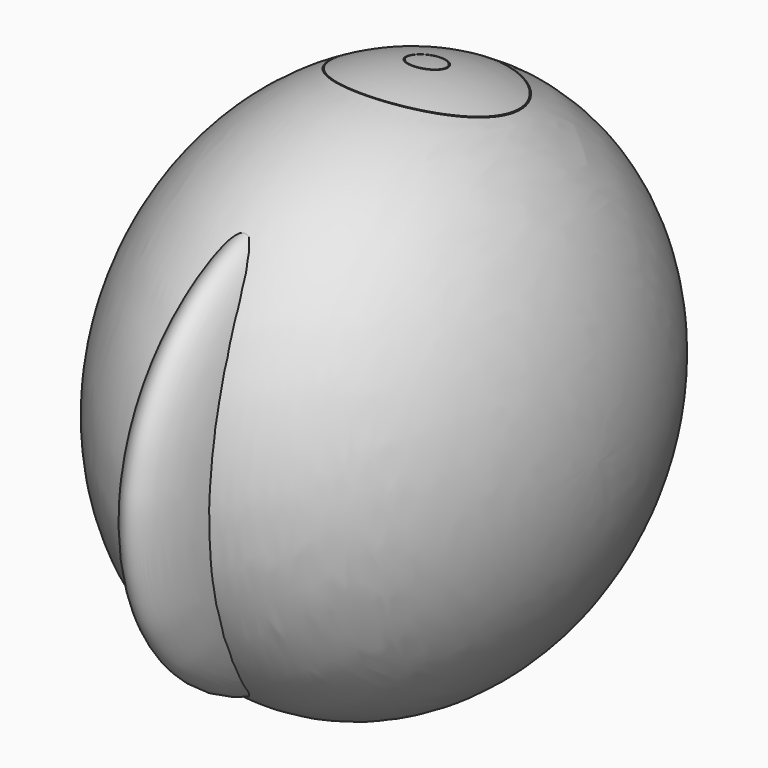
from build123d import *

# Parameters (mm, degrees)
F6_DEPTH = 250.0010001


with BuildPart() as f1:
    # F0 (on Top) → F1 (revolve)
    with BuildSketch(Plane.XY):
        with BuildLine():
            Line((0, 0), (50, 0))
            add(Edge.make_bspline(
                [(50, 0), (50, 200), (0, 200)],
                knots=[1.5707963268, 1.5707963268, 1.5707963268, 3.1415926536, 3.1415926536, 3.1415926536], degree=2, weights=[1, 0.7071067812, 1]))
            Line((0, 200), (0, 0))
        make_face()
        with BuildLine():
            Line((0, 0), (0, 200))
            add(Edge.make_bspline(
                [(0, 200), (-50, 200), (-50, 0)],
                knots=[3.1415926536, 3.1415926536, 3.1415926536, 4.7123889804, 4.7123889804, 4.7123889804], degree=2, weights=[1, 0.7071067812, 1]))
            Line((-50, 0), (0, 0))
        make_face()
    revolve(axis=Axis((53.4832403064, 0, 0), (1, 0, 0)))


with BuildPart() as f3:
    # F2 (on Top) → F3 (revolve)
    with BuildSketch(Plane.XY):
        with BuildLine():
            Line((0, 100), (200, 100))
            add(Edge.make_bspline(
                [(200, 100), (200, 350), (0, 350), (-200, 350), (-200, 100)],
                knots=[4.7123889804, 4.7123889804, 4.7123889804, 6.2831853072, 6.2831853072, 7.853981634, 7.853981634, 7.853981634], degree=2, weights=[1, 0.7071067812, 1, 0.7071067812, 1]))
            Line((-200, 100), (-175.48173666, 100))
            Line((-175.48173666, 100), (0, 100))
        make_face()
    revolve(axis=Axis((253.5901129246, 100, 0), (1, 0, 0)))


with BuildPart() as f6_tool:
    # F5 (on Top) → F6 (new body, through all)
    with BuildSketch(Plane.XY):
        with BuildLine():
            ThreePointArc((0, 226), (-76, 150), (0, 74))
            Line((0, 74), (0, 75))
            ThreePointArc((0, 75), (-75, 150), (0, 225))
            Line((0, 225), (0, 226))
        make_face()
        with BuildLine():
            Line((0, 75), (0, 74))
            ThreePointArc((0, 74), (53.7401153702, 96.2598846298), (76, 150))
            ThreePointArc((76, 150), (53.7401153702, 203.7401153702), (0, 226))
            Line((0, 226), (0, 225))
            ThreePointArc((0, 225), (53.033008589, 203.033008589), (75, 150))
            ThreePointArc((75, 150), (53.033008589, 96.966991411), (0, 75))
        make_face()
        with BuildLine():
            Line((0, 134), (0, 133))
            ThreePointArc((0, 133), (12.0208152802, 137.9791847198), (17, 150))
            ThreePointArc((17, 150), (12.0208152802, 162.0208152802), (0, 167))
            Line((0, 167), (0, 166))
            ThreePointArc((0, 166), (11.313708499, 161.313708499), (16, 150))
            ThreePointArc((16, 150), (11.313708499, 138.686291501), (0, 134))
        make_face()
        with BuildLine():
            ThreePointArc((0, 167), (-17, 150), (0, 133))
            Line((0, 133), (0, 134))
            ThreePointArc((0, 134), (-16, 150), (0, 166))
            Line((0, 166), (0, 167))
        make_face()
    extrude(amount=F6_DEPTH)


with BuildPart() as f1_1:
    add(f1.part)

    # F6: cut by f6_tool
    add(f6_tool.part, mode=Mode.SUBTRACT)


with BuildPart() as f3_1:
    add(f3.part)

    # F6: cut by f6_tool
    add(f6_tool.part, mode=Mode.SUBTRACT)


solid = Compound([f1_1.part, f3_1.part])
